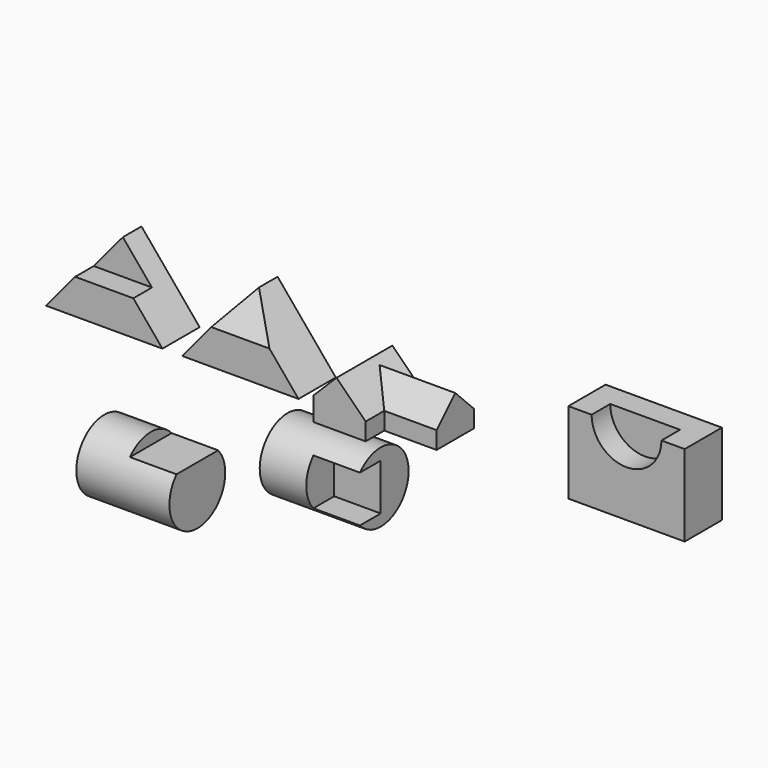
from build123d import *

# Parameters (mm, degrees)
F1_DEPTH   = 101.6
F3_DEPTH   = 50.8
F5_DEPTH   = 101.6
F6_W       = 127
F6_H       = 50.8
F7_DEPTH   = 101.6
F8_SIZE    = 50.79999
F10_DEPTH  = 101.6
F11_DEPTH  = 101.6
F11_FACE_W = 254
F11_FACE_H = 177.8
F12_DEPTH  = 50.8
F14_DEPTH  = 50.8
F16_DEPTH  = 50.8
F17_R      = 76.2
F18_DEPTH  = 203.2
F20_DEPTH  = 101.6
F23_DEPTH  = 203.2
F25_DEPTH  = 101.6
F29_DEPTH  = 76.2


# Not quite as in the source:
# - a fillet or chamfer is up to 0.001 mm smaller than in the source, because OpenCascade refuses the exact size
# - ends of sketch curves that miss each other by under 0.0002 mm in the source are joined


with BuildPart() as f1:
    # F0 (on Front) → F1 (new body)
    with BuildSketch(Plane.XZ):
        Polygon((0, 152.4), (-63.5, 76.2), (0, 76.2), (63.5, 76.2), align=None)
        Polygon((-127, 0), (0, 0), (127, 0), (63.5, 76.2), (0, 76.2), (-63.5, 76.2), align=None)
    extrude(amount=-F1_DEPTH)

    # F2 (on face) → F3 (cut)
    with BuildSketch(Plane.XZ):
        Polygon((-63.5, 76.2), (0, 76.2), (63.5, 76.2), (0, 152.4), align=None)
    extrude(amount=-F3_DEPTH, mode=Mode.SUBTRACT)


with BuildPart() as f5:
    # F4 (on Front) → F5 (new body)
    with BuildSketch(Plane.XZ):
        Polygon((233.6774150133, 76.2), (170.1774150133, 0), (424.1774150133, 0), (360.6774150133, 76.2), (297.1774150133, 76.2), align=None)
        Polygon((297.1774150133, 152.4), (233.6774150133, 76.2), (297.1774150133, 76.2), (360.6774150133, 76.2), align=None)
    extrude(amount=-F5_DEPTH)

    # F28 (on 3pt) → F29 (cut, symmetric)
    with BuildSketch(Plane.YZ.offset(297.1774150133)):
        Polygon((50.8, 152.4), (0, 152.4), (0, 76.2), align=None)
    extrude(amount=F29_DEPTH, both=True, mode=Mode.SUBTRACT)


with BuildPart() as f7:
    # F6 (on Front) → F7 (new body)
    with BuildSketch(Plane.XZ):
        Polygon((496.9945251942, 50.8), (496.9945251942, 0), (598.5945251942, 0), (598.5945251942, 50.8), (560.4945251942, 88.9), (547.7945251942, 101.6), align=None)
        Polygon((560.4945251942, 88.9), (598.5945251942, 50.8), (725.5945251942, 50.8), (725.5945251942, 88.9), align=None)
        with Locations((662.0945251942, 25.4)):
            Rectangle(F6_W, F6_H)
    extrude(amount=-F7_DEPTH)

    # F8 (size 50.8 in the source; OpenCascade refuses exactly that, so slightly less here)
    f8_edges = [f7.edges().sort_by_distance(p)[0] for p in [
        (643.044525, 0, 88.9),
        (643.044525, 101.6, 88.9),
    ]]
    chamfer(f8_edges, length=F8_SIZE)

    # F15 (on face) → F16 (join)
    with BuildSketch(Plane.XZ):
        Polygon((611.2945251942, 0), (611.2945251942, 38.1), (560.4945251942, 88.9), (547.7945251942, 101.6), (496.9945251942, 50.8), (496.9945251942, 0), align=None)
    extrude(amount=F16_DEPTH)


with BuildPart() as f10:
    # F9 (on Front) → F10 (new body)
    with BuildSketch(Plane.XZ):
        with BuildLine():
            Line((1013.2026672363, 177.8), (1013.2026672363, 0))
            Line((1013.2026672363, 0), (1267.2026672363, 0))
            Line((1267.2026672363, 0), (1267.2026672363, 177.8))
            Line((1267.2026672363, 177.8), (1216.4026672363, 177.8))
            ThreePointArc((1216.4026672363, 177.8), (1140.2026672363, 101.6), (1064.0026672363, 177.8))
            Line((1064.0026672363, 177.8), (1013.2026672363, 177.8))
        make_face()
    extrude(amount=-F10_DEPTH)

    # F9 (on Front) → F11 (join)
    with BuildSketch(Plane.XZ):
        with BuildLine():
            Line((1013.2026672363, 177.8), (1013.2026672363, 0))
            Line((1013.2026672363, 0), (1267.2026672363, 0))
            Line((1267.2026672363, 0), (1267.2026672363, 177.8))
            Line((1267.2026672363, 177.8), (1216.4026672363, 177.8))
            ThreePointArc((1216.4026672363, 177.8), (1140.2026672363, 101.6), (1064.0026672363, 177.8))
            Line((1064.0026672363, 177.8), (1013.2026672363, 177.8))
        make_face()
        with BuildLine():
            Line((1216.4026672363, 177.8), (1064.0026672363, 177.8))
            ThreePointArc((1064.0026672363, 177.8), (1140.2026672363, 101.6), (1216.4026672363, 177.8))
        make_face()
    extrude(amount=-F11_DEPTH)

    # F9 (on Front) + F11_face (on face) → F12 (cut)
    with BuildSketch(Plane.XZ):
        with BuildLine():
            Line((1013.2026672363, 177.8), (1013.2026672363, 0))
            Line((1013.2026672363, 0), (1267.2026672363, 0))
            Line((1267.2026672363, 0), (1267.2026672363, 177.8))
            Line((1267.2026672363, 177.8), (1216.4026672363, 177.8))
            ThreePointArc((1216.4026672363, 177.8), (1140.2026672363, 101.6), (1064.0026672363, 177.8))
            Line((1064.0026672363, 177.8), (1013.2026672363, 177.8))
        make_face()
        with BuildLine():
            Line((1216.4026672363, 177.8), (1064.0026672363, 177.8))
            ThreePointArc((1064.0026672363, 177.8), (1140.2026672363, 101.6), (1216.4026672363, 177.8))
        make_face()
    with BuildSketch(Plane(origin=(1140.2026672363, 0, 88.9), x_dir=(1, 0, 0), z_dir=(0, -1, 0))):
        Rectangle(F11_FACE_W, F11_FACE_H)
    extrude(amount=-F12_DEPTH, mode=Mode.SUBTRACT)

    # F13 (on face) → F14 (join)
    with BuildSketch(Plane.XZ.offset(-50.8)):
        with BuildLine():
            Line((1013.2026672363, 177.8), (1013.2026672363, 0))
            Line((1013.2026672363, 0), (1267.2026672363, 0))
            Line((1267.2026672363, 0), (1267.2026672363, 177.8))
            Line((1267.2026672363, 177.8), (1216.4026672363, 177.8))
            ThreePointArc((1216.4026672363, 177.8), (1140.2026672363, 101.6), (1064.0026672363, 177.8))
            Line((1064.0026672363, 177.8), (1013.2026672363, 177.8))
        make_face()
    extrude(amount=F14_DEPTH)


with BuildPart() as f18:
    # F17 (on Right) → F18 (new body)
    with BuildSketch(Plane.YZ):
        with Locations((0, -244.4293797016)):
            Circle(F17_R)
    extrude(amount=F18_DEPTH)

    # F19 (on face) → F20 (cut)
    with BuildSketch(Plane.YZ.offset(203.2)):
        with BuildLine():
            Line((-56.7961266285, -193.6293797016), (0, -193.6293797016))
            Line((0, -193.6293797016), (56.7961266285, -193.6293797016))
            ThreePointArc((56.7961266285, -193.6293797016), (0, -168.2293797016), (-56.7961266285, -193.6293797016))
        make_face()
    extrude(amount=-F20_DEPTH, mode=Mode.SUBTRACT)


with BuildPart() as f23:
    # F22 (on offset) → F23 (new body)
    with BuildSketch(Plane.YZ.offset(241.3)):
        with BuildLine():
            Line((198.8355070353, -192.6963732958), (142.0393804068, -192.6963732958))
            ThreePointArc((142.0393804068, -192.6963732958), (122.6355070353, -243.4963732958), (142.0393804068, -294.2963732958))
            Line((142.0393804068, -294.2963732958), (198.8355070353, -294.2963732958))
            Line((198.8355070353, -294.2963732958), (198.8355070353, -243.4963732958))
            Line((198.8355070353, -243.4963732958), (198.8355070353, -192.6963732958))
        make_face()
        with BuildLine():
            ThreePointArc((142.0393804068, -294.2963732958), (226.025350276, -314.6803070487), (275.0355070353, -243.4963732958))
            ThreePointArc((275.0355070353, -243.4963732958), (226.025350276, -172.3124395428), (142.0393804068, -192.6963732958))
            Line((142.0393804068, -192.6963732958), (198.8355070353, -192.6963732958))
            Line((198.8355070353, -192.6963732958), (198.8355070353, -243.4963732958))
            Line((198.8355070353, -243.4963732958), (198.8355070353, -294.2963732958))
            Line((198.8355070353, -294.2963732958), (142.0393804068, -294.2963732958))
        make_face()
    extrude(amount=F23_DEPTH)

    # F24 (on face) → F25 (cut)
    with BuildSketch(Plane.YZ.offset(444.5)):
        with BuildLine():
            Line((198.8355070353, -294.2963732958), (198.8355070353, -243.4963732958))
            Line((198.8355070353, -243.4963732958), (198.8355070353, -192.6963732958))
            Line((198.8355070353, -192.6963732958), (142.0393804068, -192.6963732958))
            ThreePointArc((142.0393804068, -192.6963732958), (122.6355070353, -243.4963732958), (142.0393804068, -294.2963732958))
            Line((142.0393804068, -294.2963732958), (198.8355070353, -294.2963732958))
        make_face()
    extrude(amount=-F25_DEPTH, mode=Mode.SUBTRACT)


solid = Compound([f1.part, f5.part, f7.part, f10.part, f18.part, f23.part])
